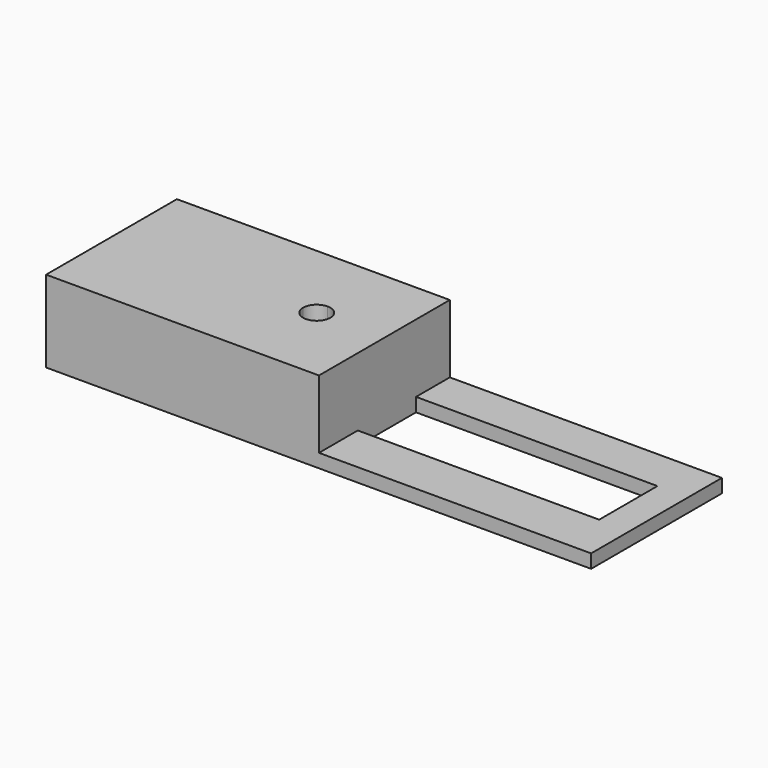
from build123d import *

# Parameters (mm, degrees)
F1_DEPTH = 6
F2_DEPTH = 1


with BuildPart() as f1:
    # F0 (on Top) → F1 (new body)
    with BuildSketch(Plane.XY):
        Polygon((-25, 0), (-19.9713055044, 0), (-19.9713055044, 3.5559397656), (-24.9629596584, 3.5559397656), align=None)
        Polygon((-40, 0), (-25, 0), (-24.9629596584, 3.5559397656), (-40, 3.5559397656), align=None)
        with BuildLine():
            Line((-24.9629596584, 3.5559397656), (-19.9713055044, 3.5559397656))
            Line((-19.9713055044, 3.5559397656), (-19.9713055044, 6))
            Line((-19.9713055044, 6), (-23.9375011772, 6))
            ThreePointArc((-23.9375011772, 6), (-24.2340866143, 5.2892201799), (-24.9479170826, 5.000054247))
            Line((-24.9479170826, 5.000054247), (-24.9629596584, 3.5559397656))
        make_face()
        with BuildLine():
            Line((-19.9713055044, 8.8996905833), (-19.9713055044, 12))
            Line((-19.9713055044, 12), (-24.9375011772, 12))
            Line((-24.9375011772, 12), (-24.9375011772, 7))
            ThreePointArc((-24.9375011772, 7), (-24.230394396, 6.7071067812), (-23.9375011772, 6))
            Line((-23.9375011772, 6), (-19.9713055044, 6))
            Line((-19.9713055044, 6), (-19.9713055044, 8.8996905833))
        make_face()
        with BuildLine():
            Line((-40, 3.5559397656), (-24.9629596584, 3.5559397656))
            Line((-24.9629596584, 3.5559397656), (-24.9479170826, 5.000054247))
            ThreePointArc((-24.9479170826, 5.000054247), (-25.6482809973, 5.2965854371), (-25.9375011772, 6))
            Line((-25.9375011772, 6), (-40, 6))
            Line((-40, 6), (-40, 3.5559397656))
        make_face()
        with BuildLine():
            Line((-24.9375011772, 7), (-24.9375011772, 12))
            Line((-24.9375011772, 12), (-40, 12))
            Line((-40, 12), (-40, 6))
            Line((-40, 6), (-25.9375011772, 6))
            ThreePointArc((-25.9375011772, 6), (-25.6446079584, 6.7071067812), (-24.9375011772, 7))
        make_face()
    extrude(amount=F1_DEPTH)

    # F0 (on Top) → F2 (join)
    with BuildSketch(Plane.XY):
        Polygon((-19.9713055044, 0), (0, 0), (0, 12), (-19.9713055044, 12), (-19.9713055044, 8.8996905833), (-2.2525554523, 8.8996905833), (-2.2525554523, 3.5559397656), (-19.9713055044, 3.5559397656), align=None)
    extrude(amount=F2_DEPTH)


solid = f1.part
